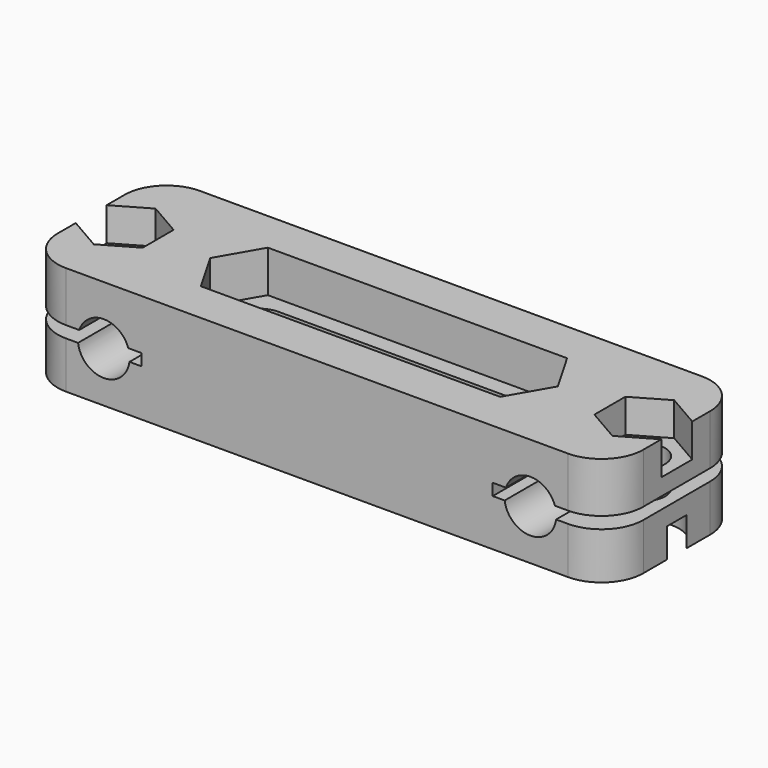
from build123d import *

# Parameters (mm, degrees)
F0_W      = 70
F0_H      = 20
F1_DEPTH  = 6.5
F4_DEPTH  = 4
F5_R      = 2.6
F6_DEPTH  = 13.001
F7_DEPTH  = 13.001
F8_W      = 14
F8_H      = 1.4
F9_DEPTH  = 20.001
F11_R     = 5
F10_R     = 3.1
F12_DEPTH = 20.001
F13_R     = 4.25
F14_DEPTH = 3.5
F16_DEPTH = 5


with BuildPart() as f1:
    # F0 (on Top) → F1 (new body, symmetric)
    with BuildSketch(Plane.XY):
        Rectangle(F0_W, F0_H)
    extrude(amount=F1_DEPTH, both=True)

    # F3 (on face) → F4 (cut)
    with BuildSketch(Plane.XY.offset(6.5)):
        Polygon((-31, -4.6188021535), (-27, -2.3094010768), (-27, 2.3094010768), (-31, 4.6188021535), (-35, 2.3094010768), (-35, -2.3094010768), align=None)
        Polygon((35, -2.3094010768), (35, 2.3094010768), (31, 4.6188021535), (27, 2.3094010768), (27, -2.3094010768), (31, -4.6188021535), align=None)
    extrude(amount=-F4_DEPTH, mode=Mode.SUBTRACT)

    # F5 (on face) → F6 (cut, through all)
    with BuildSketch(Plane.XY.offset(6.5)):
        with Locations((-31, 0)):
            Circle(F5_R)
        with Locations((31, 0)):
            Circle(F5_R)
    extrude(amount=-F6_DEPTH, mode=Mode.SUBTRACT)

    # F2 (on face) → F7 (cut, through all)
    with BuildSketch(Plane.XY.offset(6.5)):
        with BuildLine():
            Line((-15, -3), (15, -3))
            ThreePointArc((15, -3), (18, 0), (15, 3))
            Line((15, 3), (-15, 3))
            ThreePointArc((-15, 3), (-18, 0), (-15, -3))
        make_face()
    extrude(amount=-F7_DEPTH, mode=Mode.SUBTRACT)

    # F8 (on face) → F9 (cut, through all)
    with BuildSketch(Plane.XZ.offset(10)):
        with Locations((-28, -0.2)):
            Rectangle(F8_W, F8_H)
        with Locations((28, -0.2)):
            Rectangle(F8_W, F8_H)
    extrude(amount=-F9_DEPTH, mode=Mode.SUBTRACT)

    # F11
    f11_edges = [f1.edges().sort_by_distance(p)[0] for p in [
        (35, 10, 3.5),
        (35, 10, -3.7),
        (35, -10, 3.5),
        (35, -10, -3.7),
        (-35, -10, -3.7),
        (-35, -10, 3.5),
        (-35, 10, 3.5),
        (-35, 10, -3.7),
    ]]
    fillet(f11_edges, radius=F11_R)

    # F10 (on face) → F12 (cut, through all)
    with BuildSketch(Plane.XZ.offset(10)):
        with Locations((-25.5, -0.5)):
            Circle(F10_R)
        with Locations((25.5, -0.5)):
            Circle(F10_R)
    extrude(amount=-F12_DEPTH, mode=Mode.SUBTRACT)

    # F13 (on face) → F14 (cut)
    with BuildSketch(Plane(origin=(0, 0, -6.5), x_dir=(1, 0, 0), z_dir=(0, 0, -1))):
        with Locations((31, 0)):
            Circle(F13_R)
        with Locations((-31, 0)):
            Circle(F13_R)
    extrude(amount=-F14_DEPTH, mode=Mode.SUBTRACT)

    # F15 (on face) → F16 (cut)
    with BuildSketch(Plane.XY.offset(6.5)):
        Polygon((-17.8867513459, -5), (-12.1132486541, -5), (-9.2264973081, 0), (-12.1132486541, 5), (-17.8867513459, 5), (-20.7735026919, 0), align=None)
        Polygon((-9.2264973081, 0), (-12.1132486541, -5), (12.1132486541, -5), (9.2264973081, 0), (12.1132486541, 5), (-12.1132486541, 5), align=None)
        Polygon((9.2264973081, 0), (12.1132486541, -5), (17.8867513459, -5), (20.7735026919, 0), (17.8867513459, 5), (12.1132486541, 5), align=None)
    extrude(amount=-F16_DEPTH, mode=Mode.SUBTRACT)


solid = f1.part
